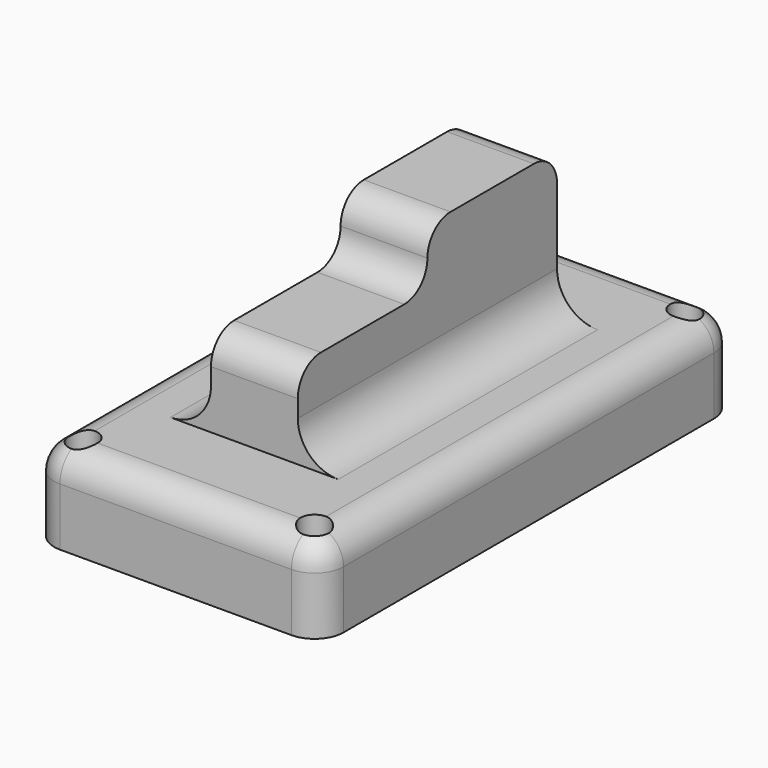
from build123d import *

# Parameters (mm, degrees)
F0_R         = 2.5
F1_DEPTH     = 15
F0_W         = 15
F0_H         = 28
F2_DEPTH     = 40
F3_DEPTH     = 30
F4_T1_DEPTH  = 15
F4_T3_DEPTH  = 40
F4_T5_DEPTH  = 80
F4_T8_ANGLE  = 90
F4_T10_ANGLE = 90
F4_T12_ANGLE = 90
F4_T14_ANGLE = 90
F5_R         = 7


# Not quite as in the source:
# - a fillet or chamfer that OpenCascade refuses, or shapes differently, is made with other operations: its cross-section is extruded or revolved along the edge and cut away or added


with BuildPart() as f1:
    # F0 (on Top) → F1 (new body)
    with BuildSketch(Plane.XY):
        with BuildLine():
            ThreePointArc((-25, -40), (-23.5355339059, -43.5355339059), (-20, -45))
            Line((-20, -45), (20, -45))
            ThreePointArc((20, -45), (23.5355339059, -43.5355339059), (25, -40))
            Line((25, -40), (25, 40))
            ThreePointArc((25, 40), (23.5355339059, 43.5355339059), (20, 45))
            Line((20, 45), (-20, 45))
            ThreePointArc((-20, 45), (-23.5355339059, 43.5355339059), (-25, 40))
            Line((-25, 40), (-25, -40))
        make_face()
        with Locations((-20, -40)):
            Circle(F0_R, mode=Mode.SUBTRACT)
        with Locations((20, -40)):
            Circle(F0_R, mode=Mode.SUBTRACT)
        with Locations((-20, 40)):
            Circle(F0_R, mode=Mode.SUBTRACT)
        Polygon((7.5, 28), (7.5, 0), (7.5, -28), (-7.5, -28), (-7.5, 0), (-7.5, 28), align=None, mode=Mode.SUBTRACT)
        with Locations((20, 40)):
            Circle(F0_R, mode=Mode.SUBTRACT)
    extrude(amount=F1_DEPTH)

    # F0 (on Top) → F2 (join)
    with BuildSketch(Plane.XY):
        with Locations((0, 14)):
            Rectangle(F0_W, F0_H)
    extrude(amount=F2_DEPTH)

    # F0 (on Top) → F3 (join)
    with BuildSketch(Plane.XY):
        with Locations((0, -14)):
            Rectangle(F0_W, F0_H)
    extrude(amount=F3_DEPTH)

    # F4: fillet of radius 5 on 6 edges, made by hand

    # F4_s2 → F4_t1 (join)
    with BuildSketch(Plane.YZ.offset(-7.5)):
        with BuildLine():
            ThreePointArc((0, 35), (-1.4644660941, 31.4644660941), (-5, 30))
            Line((-5, 30), (0, 30))
            Line((0, 30), (0, 35))
        make_face()
    extrude(amount=F4_T1_DEPTH)

    # F4_s4 → F4_t3 (cut)
    with BuildSketch(Plane.YZ.offset(-20)):
        with BuildLine():
            ThreePointArc((0, 35), (1.4644660941, 38.5355339059), (5, 40))
            Line((5, 40), (0, 40))
            Line((0, 40), (0, 35))
        make_face()
        with BuildLine():
            ThreePointArc((28, 35), (26.5355339059, 38.5355339059), (23, 40))
            Line((23, 40), (28, 40))
            Line((28, 40), (28, 35))
        make_face()
        with BuildLine():
            ThreePointArc((-45, 10), (-43.5355339059, 13.5355339059), (-40, 15))
            Line((-40, 15), (-45, 15))
            Line((-45, 15), (-45, 10))
        make_face()
        with BuildLine():
            ThreePointArc((-28, 25), (-26.5355339059, 28.5355339059), (-23, 30))
            Line((-23, 30), (-28, 30))
            Line((-28, 30), (-28, 25))
        make_face()
        with BuildLine():
            ThreePointArc((40, 15), (43.5355339059, 13.5355339059), (45, 10))
            Line((45, 10), (45, 15))
            Line((45, 15), (40, 15))
        make_face()
    extrude(amount=F4_T3_DEPTH, mode=Mode.SUBTRACT)

    # F4_s6 → F4_t5 (cut)
    with BuildSketch(Plane.XZ.offset(-40)):
        with BuildLine():
            ThreePointArc((-25, 10), (-23.5355339059, 13.5355339059), (-20, 15))
            Line((-20, 15), (-25, 15))
            Line((-25, 15), (-25, 10))
        make_face()
        with BuildLine():
            ThreePointArc((20, 15), (23.5355339059, 13.5355339059), (25, 10))
            Line((25, 10), (25, 15))
            Line((25, 15), (20, 15))
        make_face()
    extrude(amount=F4_T5_DEPTH, mode=Mode.SUBTRACT)

    # F4_s7 → F4_t8 (revolve, cut)
    with BuildSketch(Plane.XZ.offset(40)):
        with BuildLine():
            ThreePointArc((-25, 10), (-23.5355339059, 13.5355339059), (-20, 15))
            Line((-20, 15), (-25, 15))
            Line((-25, 15), (-25, 10))
        make_face()
    revolve(axis=Axis((-20, -40, 15), (0, 0, 1)), revolution_arc=F4_T8_ANGLE, mode=Mode.SUBTRACT)

    # F4_s9 → F4_t10 (revolve, cut)
    with BuildSketch(Plane.YZ.offset(-20)):
        with BuildLine():
            ThreePointArc((40, 15), (43.5355339059, 13.5355339059), (45, 10))
            Line((45, 10), (45, 15))
            Line((45, 15), (40, 15))
        make_face()
    revolve(axis=Axis((-20, 40, 15), (0, 0, 1)), revolution_arc=F4_T10_ANGLE, mode=Mode.SUBTRACT)

    # F4_s11 → F4_t12 (revolve, cut)
    with BuildSketch(Plane.XZ.offset(-40)):
        with BuildLine():
            ThreePointArc((20, 15), (23.5355339059, 13.5355339059), (25, 10))
            Line((25, 10), (25, 15))
            Line((25, 15), (20, 15))
        make_face()
    revolve(axis=Axis((20, 40, 15), (0, 0, 1)), revolution_arc=F4_T12_ANGLE, mode=Mode.SUBTRACT)

    # F4_s13 → F4_t14 (revolve, cut)
    with BuildSketch(Plane.YZ.offset(20)):
        with BuildLine():
            ThreePointArc((-40, 15), (-43.5355339059, 13.5355339059), (-45, 10))
            Line((-45, 10), (-45, 15))
            Line((-45, 15), (-40, 15))
        make_face()
    revolve(axis=Axis((20, -40, 15), (0, 0, 1)), revolution_arc=F4_T14_ANGLE, mode=Mode.SUBTRACT)

    # F5
    f5_edges = [f1.edges().sort_by_distance(p)[0] for p in [
        (-7.5, 0, 15),
        (7.5, 0, 15),
    ]]
    fillet(f5_edges, radius=F5_R)


solid = f1.part
